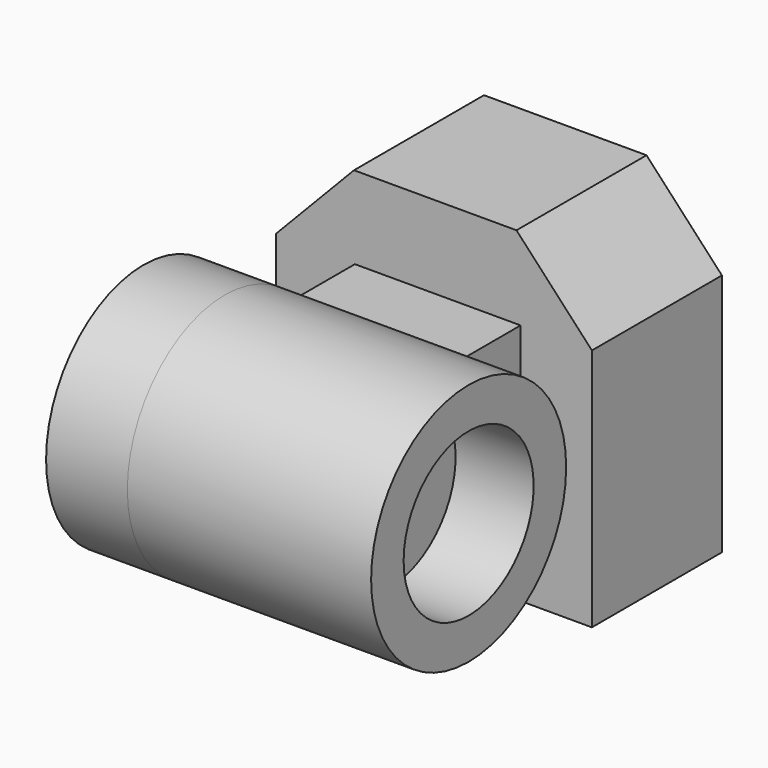
from build123d import *

# Parameters (mm, degrees)
F1_DEPTH  = 12.7
F3_DEPTH  = 12.7
F5_DEPTH  = 12.7
F7_DEPTH  = 12.7
F8_R      = 9.525
F9_DEPTH  = 19.05
F10_DEPTH = 6.35
F11_R     = 6.35
F12_DEPTH = 25.4


# Not quite as in the source:
# - a feature of the source that left no trace in its solid (it failed there, or was rolled back) is left out


with BuildPart() as f1:
    # F0 (on Front) → F1 (new body)
    with BuildSketch(Plane.XZ):
        Polygon((0, 19.05), (0, 0), (24.6888007513, 0), (24.6888007513, 19.05), (18.7959997422, 19.05), (18.7959997422, 25.4), (6.0959997422, 25.4), (6.0959997422, 19.05), align=None)
    extrude(amount=F1_DEPTH)

    # F2 (on face) → F3 (join)
    with BuildSketch(Plane.XZ.offset(12.7)):
        Polygon((6.0959997422, 25.4), (0, 19.05), (6.0959997422, 19.05), align=None)
    extrude(amount=-F3_DEPTH)

    # F4 (on face) → F5 (join)
    with BuildSketch(Plane.XZ.offset(12.7)):
        Polygon((24.6888007513, 19.05), (18.7959997422, 25.4), (18.7959997422, 19.05), align=None)
    extrude(amount=-F5_DEPTH)

    # F6 (on face) → F7 (join)
    with BuildSketch(Plane.XZ.offset(12.7)):
        Polygon((19.1160719842, 18.9619082958), (12.6412734389, 18.9619082958), (6.1664739624, 18.9619082958), (6.1664739624, 6.0123121366), (19.1160719842, 6.0123121366), align=None)
    extrude(amount=F7_DEPTH)


with BuildPart() as f9:
    # F8 (on face) → F9 (new body)
    with BuildSketch(Plane(origin=(6.1664739624, 0, 0), x_dir=(0, -1, 0), z_dir=(-1, 0, 0))):
        with Locations((25.4, 12.4871102162)):
            Circle(F8_R)
    extrude(amount=-F9_DEPTH)


with BuildPart() as f10:
    # F10 (new): a face of the model
    f10_faces = [f9.part.faces().sort_by_distance(p)[0] for p in [
        (6.1664739624, -25.4, 12.4871102162),
    ]]
    extrude(f10_faces, amount=F10_DEPTH)


with BuildPart() as f12_tool:
    # F11 (on face) → F12 (new body)
    with BuildSketch(Plane(origin=(-0.1835260376, 0, 0), x_dir=(0, -1, 0), z_dir=(-1, 0, 0))):
        with Locations((25.4, 12.4871102162)):
            Circle(F11_R)
    extrude(amount=-F12_DEPTH)


with BuildPart() as f9_1:
    add(f9.part)

    # F12: cut by f12_tool
    add(f12_tool.part, mode=Mode.SUBTRACT)


with BuildPart() as f10_1:
    add(f10.part)

    # F12: cut by f12_tool
    add(f12_tool.part, mode=Mode.SUBTRACT)


solid = Compound([f1.part, f9_1.part, f10_1.part])
